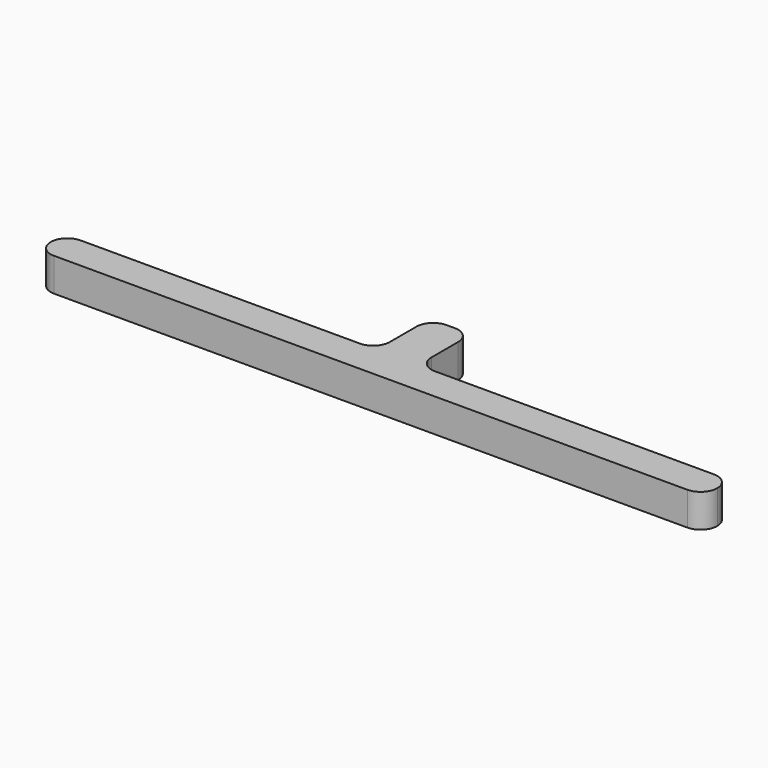
from build123d import *

# Parameters (mm, degrees)
F0_W     = 5
F0_H     = 8
F1_DEPTH = 4
F2_R     = 1.99999


# Not quite as in the source:
# - a fillet or chamfer is up to 0.001 mm smaller than in the source, because OpenCascade refuses the exact size


with BuildPart() as f1:
    # F0 (on Top) → F1 (new body)
    with BuildSketch(Plane.XY):
        Polygon((-2.5, 2), (-40, 2), (-40, -2), (40, -2), (40, 2), (2.5, 2), align=None)
        with Locations((0, 6)):
            Rectangle(F0_W, F0_H)
    extrude(amount=F1_DEPTH)

    # F2 (radius 2 in the source; OpenCascade refuses exactly that, so slightly less here)
    f2_edges = [f1.edges().sort_by_distance(p)[0] for p in [
        (-40, -2, 2),
        (40, -2, 2),
        (40, 2, 2),
        (-40, 2, 2),
        (-2.5, 10, 2),
        (2.5, 10, 2),
        (-2.5, 2, 2),
        (2.5, 2, 2),
    ]]
    fillet(f2_edges, radius=F2_R)


solid = f1.part
